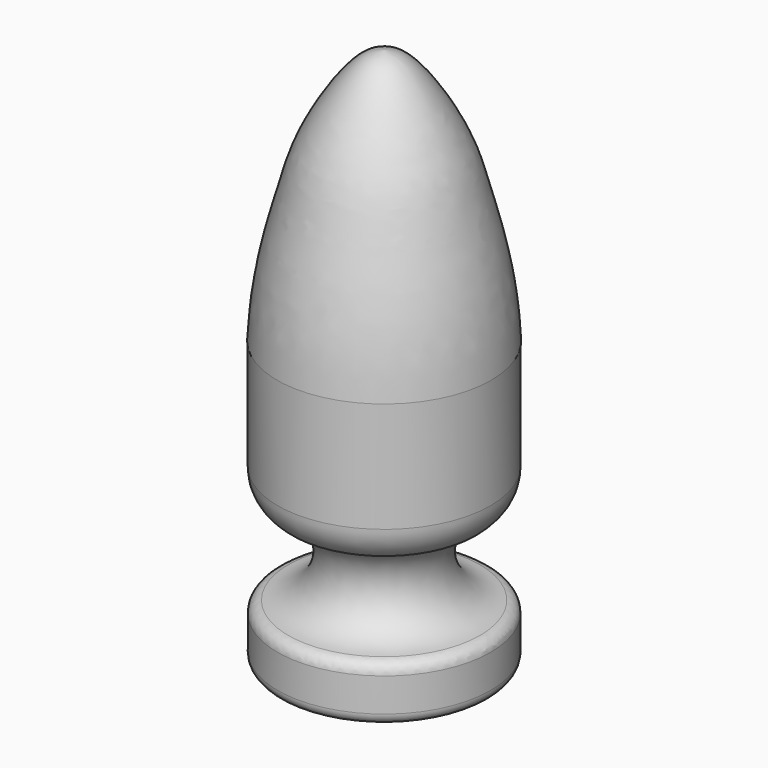
from build123d import *

# Parameters (mm, degrees)
F2_R = 2


# Not quite as in the source:
# - a fillet or chamfer that OpenCascade refuses, or shapes differently, is made with other operations: its cross-section is extruded or revolved along the edge and cut away or added


with BuildPart() as f1:
    # F0 (on Front) → F1 (revolve)
    with BuildSketch(Plane.XZ):
        with BuildLine():
            Line((18.000271342, 25.0001516185), (18.1012638153, 24.9997436393))
            add(Edge.make_bspline(
                [(18.1012638153, 24.9997436393), (17.6719067295, 35.095470957), (14.2496345804, 46.7589173288), (12.2347602329, 54.7595156146), (7.9244531632, 62.8468989209), (3.3477119391, 68.6841172693), (1.1088911486, 69.6972383356), (-0.7046223968, 69.9807515456)],
                knots=[0, 0, 0, 0, 0.3127125194, 0.4947905771, 0.691957332, 0.8656901327, 1, 1, 1, 1], degree=3))
            Line((-0.7046223968, 69.9807515456), (-0.7046223968, 25.0757137578))
            Line((-0.7046223968, 25.0757137578), (18.000271342, 25.0757137578))
            Line((18.000271342, 25.0757137578), (18.000271342, 25.0001516185))
        make_face()
        with BuildLine():
            Line((18.000271342, -0.0002563607), (18.000271342, 25.0001516185))
            Line((18.000271342, 25.0001516185), (-0.7046223968, 25.0757137578))
            Line((-0.7046223968, 25.0757137578), (-0.7046223968, 0))
            Line((-0.7046223968, 0), (-0.7046223968, -0.0002563607))
            Line((-0.7046223968, -0.0002563607), (15.250271342, -0.0002563607))
            ThreePointArc((15.250271342, -0.0002563607), (16.625271342, 0.1247436393), (18.000271342, -0.0002563607))
        make_face()
        Polygon((-0.7046223968, 25.0757137578), (18.000271342, 25.0001516185), (18.000271342, 25.0757137578), align=None)
        with BuildLine():
            Line((15.250271342, -0.0002563607), (18.000271342, -0.0002563607))
            ThreePointArc((18.000271342, -0.0002563607), (16.625271342, 0.1247436393), (15.250271342, -0.0002563607))
        make_face()
        with BuildLine():
            ThreePointArc((18.000271342, -15.0002563607), (9.125271342, -8.8752563607), (15.250271342, -0.0002563607))
            Line((15.250271342, -0.0002563607), (-0.7046223968, -0.0002563607))
            Line((-0.7046223968, -0.0002563607), (-0.7046223968, -25.0002563607))
            Line((-0.7046223968, -25.0002563607), (18.000271342, -25.0002563607))
            Line((18.000271342, -25.0002563607), (18.000271342, -15.0002563607))
        make_face()
    revolve(axis=Axis((-0.7046223968, 0, 47.5282326517), (0, 0, -1)))

    # F2
    f2_edges = [f1.edges().sort_by_distance(p)[0] for p in [
        (-19.409516, 0, -15.000256),
        (-19.409516, 0, -25.000256),
    ]]
    fillet(f2_edges, radius=F2_R)

    # F3: fillet of radius 7 on 1 edges, made by hand

    # F3_s1 → F3_t2 (revolve, cut)
    with BuildSketch(Plane.XZ):
        with BuildLine():
            ThreePointArc((15.250271342, -0.0002563607), (17.275221541, 2.4594740932), (18.000271342, 5.5618925047))
            Line((18.000271342, 5.5618925047), (18.000271342, -0.0002563607))
            Line((18.000271342, -0.0002563607), (15.250271342, -0.0002563607))
        make_face()
    revolve(axis=Axis((-0.7046223968, 0, -0.0002563607), (0, 0, -1)), mode=Mode.SUBTRACT)


solid = f1.part
